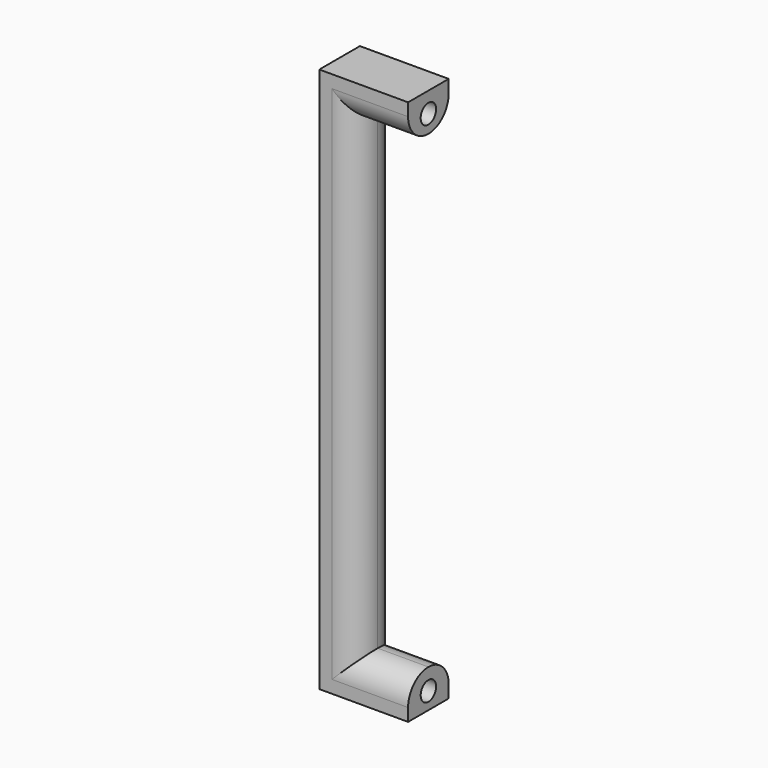
from build123d import *

# Parameters (mm, degrees)
F1_DEPTH = 12.7
F2_R     = 6.34999
F3_R     = 6.34999
F4_DEPTH = 3.175
F6_D     = 4.826
F6_DEPTH = 14.224
F6_TIP   = 1.4498766737
F8_D     = 4.826
F8_DEPTH = 14.224
F8_TIP   = 1.4498766737


# Not quite as in the source:
# - a fillet or chamfer is up to 0.001 mm smaller than in the source, because OpenCascade refuses the exact size


with BuildPart() as f1:
    # F0 (on Front) → F1 (new body)
    with BuildSketch(Plane.XZ):
        Polygon((12.7, 64.008), (12.7, 68.2625), (-12.7, 68.2625), (-12.7, -68.2625), (12.7, -68.2625), (12.7, -64.008), (12.7, -58.7375), (0, -58.7375), (0, 58.7375), (12.7, 58.7375), align=None)
    extrude(amount=F1_DEPTH)

    # F2 (radius 6.35 in the source; OpenCascade refuses exactly that, so slightly less here)
    f2_edges = [f1.edges().sort_by_distance(p)[0] for p in [
        (0, -12.7, 0),
        (0, 0, 0),
    ]]
    fillet(f2_edges, radius=F2_R)

    # F3 (radius 6.35 in the source; OpenCascade refuses exactly that, so slightly less here)
    f3_edges = [f1.edges().sort_by_distance(p)[0] for p in [
        (6.35, -12.7, 58.7375),
        (6.35, 0, 58.7375),
        (6.35, -12.7, -58.7375),
        (6.35, 0, -58.7375),
    ]]
    fillet(f3_edges, radius=F3_R)

    # F4 (cut): a face of the model
    f4_faces = [f1.faces().sort_by_distance(p)[0] for p in [
        (-12.7, -6.35, 0),
    ]]
    extrude(f4_faces, amount=-F4_DEPTH, mode=Mode.SUBTRACT)

    # F6
    with Locations(Plane.YZ.offset(12.7)):
        with Locations((-6.35, 63.1825)):
            Hole(F6_D / 2, depth=F6_DEPTH)
            with Locations((0, 0, -(F6_DEPTH + F6_TIP / 2))):  # 118° drill point
                Cone(0, F6_D / 2, F6_TIP, mode=Mode.SUBTRACT)

    # F8
    with Locations(Plane.YZ.offset(12.7)):
        with Locations((-6.35, -64.008)):
            Hole(F8_D / 2, depth=F8_DEPTH)
            with Locations((0, 0, -(F8_DEPTH + F8_TIP / 2))):  # 118° drill point
                Cone(0, F8_D / 2, F8_TIP, mode=Mode.SUBTRACT)


solid = f1.part
